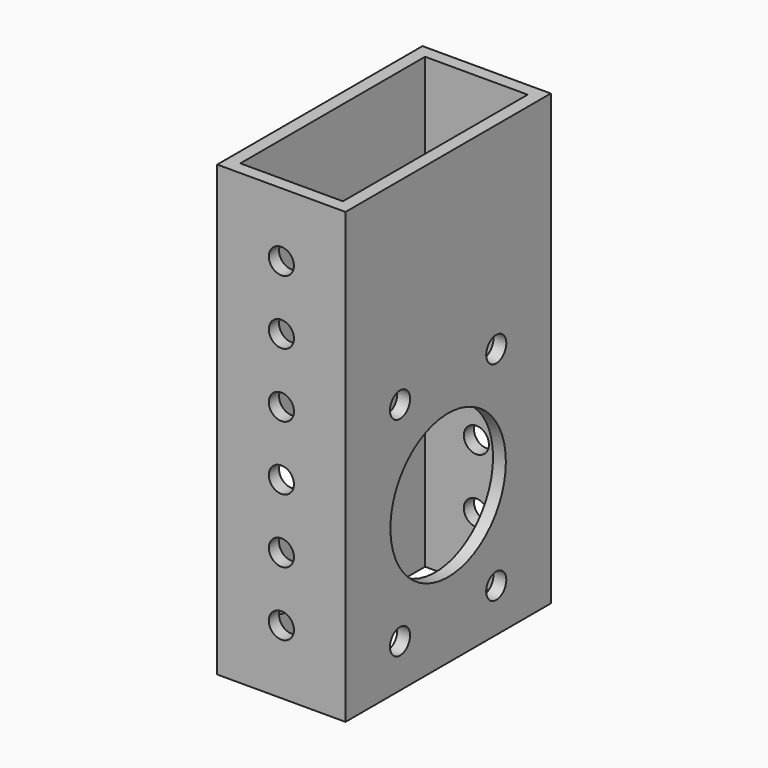
from build123d import *

# Parameters (mm, degrees)
F0_W     = 25.4
F0_H     = 50.8
F0_W_2   = 20.32
F0_H_2   = 45.72
F1_DEPTH = 88.9
F2_R     = 14.2875
F3_DEPTH = 50.8
F4_R     = 2.4892
F5_DEPTH = 25.401
F6_R     = 2.4892
F7_DEPTH = 50.801


# Not quite as in the source:
# - a feature names something its author has since deleted; it is built from what else it names


with BuildPart() as f1:
    # F0 (on Top) → F1 (new body)
    with BuildSketch(Plane.XY):
        with Locations((12.7, -25.4)):
            Rectangle(F0_W, F0_H)
        with Locations((12.7, -25.4)):
            Rectangle(F0_W_2, F0_H_2, mode=Mode.SUBTRACT)
    extrude(amount=F1_DEPTH)

    # F2 (on face) → F3 (cut)
    with BuildSketch(Plane.YZ.offset(25.4)):
        with Locations((-25.4, 29.21)):
            Circle(F2_R)
    extrude(amount=-F3_DEPTH, mode=Mode.SUBTRACT)

    # F4 (on face) → F5 (cut, through all)
    with BuildSketch(Plane.YZ.offset(25.4)):
        with Locations((-13.49375, 49.8322299276)):
            Circle(F4_R)
        with Locations((-13.49375, 8.5877700724)):
            Circle(F4_R)
        with Locations((-37.30625, 8.5877700724)):
            Circle(F4_R)
        with Locations((-37.30625, 49.8322299276)):
            Circle(F4_R)
    extrude(amount=-F5_DEPTH, mode=Mode.SUBTRACT)

    # F6 (on face) → F7 (cut, through all)
    with BuildSketch(Plane.XZ.offset(50.8)):
        with Locations((12.7, 12.7)):
            Circle(F6_R)
        with Locations((12.7, 25.4)):
            Circle(F6_R)
        with Locations((12.7, 38.1)):
            Circle(F6_R)
        with Locations((12.7, 50.8)):
            Circle(F6_R)
        with Locations((12.7, 63.5)):
            Circle(F6_R)
        with Locations((12.7, 76.2)):
            Circle(F6_R)
    extrude(amount=-F7_DEPTH, mode=Mode.SUBTRACT)


solid = f1.part
